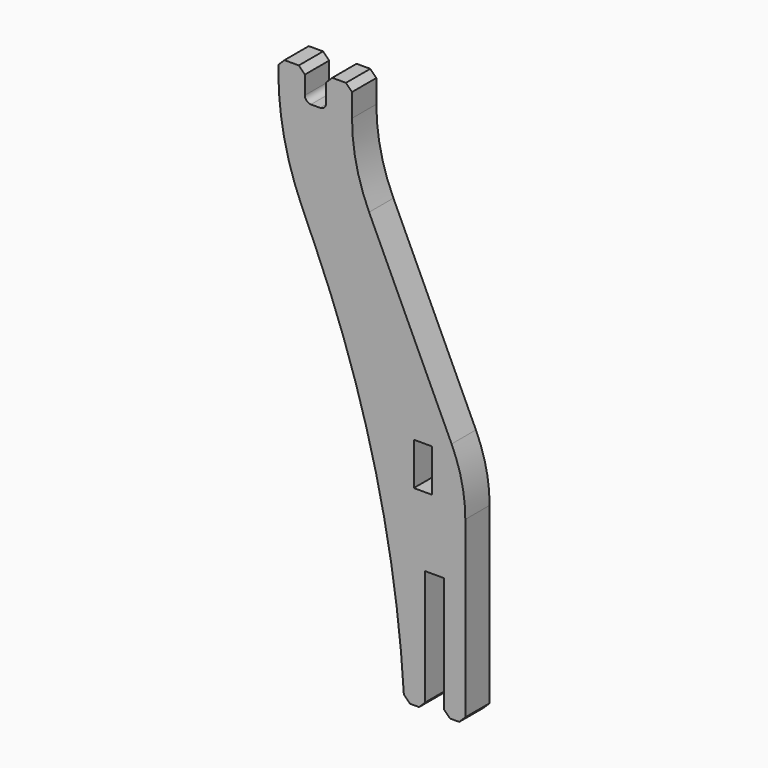
from build123d import *

# Parameters (mm, degrees)
F0_W        = 7.62
F0_H        = 17.78
F1_DEPTH    = 12.7
F2_SIZE     = 2.54
F3_R        = 61.3177298103
F4_R        = 76.3155057079
F5_R        = 114.0325409017
F6_T1_DEPTH = 12.7


# Not quite as in the source:
# - a fillet or chamfer that OpenCascade refuses, or shapes differently, is made with other operations: its cross-section is extruded or revolved along the edge and cut away or added


with BuildPart() as f1:
    # F0 (on Front) → F1 (new body)
    with BuildSketch(Plane.XZ):
        with BuildLine():
            Line((-43.3897525072, 184.0122990829), (-43.3897525072, 154.9135648233))
            Line((-43.3897525072, 154.9135648233), (-12.6282460988, 154.9135648233))
            Line((-12.6282460988, 154.9135648233), (-12.6282460988, 184.0122990829))
            Line((-12.6282460988, 184.0122990829), (-23.4354074901, 184.0122990829))
            Line((-23.4354074901, 184.0122990829), (-23.4354074901, 173.8522990829))
            ThreePointArc((-23.4354074901, 173.8522990829), (-24.1793562659, 172.0562478587), (-25.9754074901, 171.3122990829))
            Line((-25.9754074901, 171.3122990829), (-29.7854074901, 171.3122990829))
            ThreePointArc((-29.7854074901, 171.3122990829), (-31.5814587143, 172.0562478587), (-32.3254074901, 173.8522990829))
            Line((-32.3254074901, 173.8522990829), (-32.3254074901, 184.0122990829))
            Line((-32.3254074901, 184.0122990829), (-43.3897525072, 184.0122990829))
        make_face()
        Polygon((-43.3897525072, 154.9135648233), (9.0125808752, 35.5335648233), (34.6665808752, 35.5335648233), (34.6665808752, 53.3135648233), (-12.6282460988, 154.9135648233), align=None)
        with Locations((16.9659831101, 53.1658351564)):
            Rectangle(F0_W, F0_H, mode=Mode.SUBTRACT)
        Polygon((34.6665808752, 35.5335648233), (9.0125808752, 35.5335648233), (9.0125808752, -35.5335648233), (17.9025808752, -35.5335648233), (17.9025808752, 15.2664351767), (25.7765808752, 15.2664351767), (25.7765808752, -35.5335648233), (34.6665808752, -35.5335648233), align=None)
    extrude(amount=F1_DEPTH)

    # F2
    f2_edges = [f1.edges().sort_by_distance(p)[0] for p in [
        (-32.325407, -6.35, 184.012299),
        (-23.435407, -6.35, 184.012299),
        (-12.628246, -6.35, 184.012299),
        (-43.389753, -6.35, 184.012299),
        (17.902581, -6.35, -35.533565),
        (25.776581, -6.35, -35.533565),
        (34.666581, -6.35, -35.533565),
        (9.012581, -6.35, -35.533565),
    ]]
    chamfer(f2_edges, length=F2_SIZE)

    # F3
    f3_edges = [f1.edges().sort_by_distance(p)[0] for p in [
        (34.666581, -6.35, 53.313565),
    ]]
    fillet(f3_edges, radius=F3_R)

    # F4
    f4_edges = [f1.edges().sort_by_distance(p)[0] for p in [
        (-12.628246, -6.35, 154.913565),
    ]]
    fillet(f4_edges, radius=F4_R)

    # F5
    f5_edges = [f1.edges().sort_by_distance(p)[0] for p in [
        (-43.389753, -6.35, 154.913565),
    ]]
    fillet(f5_edges, radius=F5_R)

    # F6: fillet of radius 446.1798259809 on 1 edges, made by hand

    # F6_s2 → F6_t1 (join)
    with BuildSketch(Plane.XZ):
        with BuildLine():
            ThreePointArc((-27.8005344067, 119.3990994032), (-2.6481597508, 44.8323374579), (9.0125808752, -32.9935648233))
            Line((9.0125808752, -32.9935648233), (9.0125808752, 35.5335648233))
            Line((9.0125808752, 35.5335648233), (-27.8005344067, 119.3990994032))
        make_face()
    extrude(amount=F6_T1_DEPTH)


solid = f1.part
